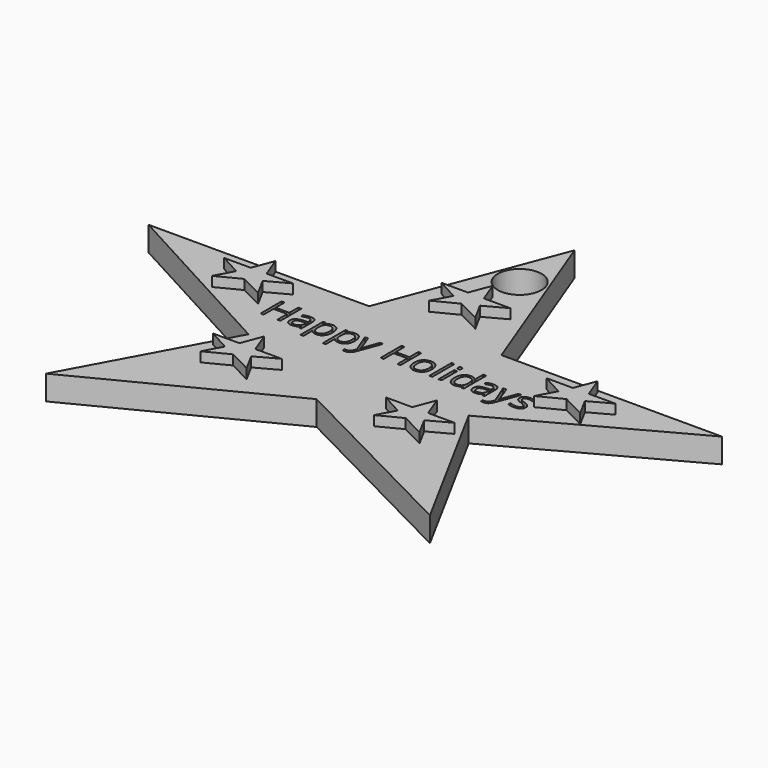
from build123d import *

# Parameters (mm, degrees)
F1_DEPTH     = 5
F2_TEXT_SIZE = 7.4632064853
F3_DEPTH     = 2.5
F4_R         = 4.4811489531
F5_DEPTH     = 25
F7_DEPTH     = 7


# Not quite as in the source:
# - Text() gives the source's letters only with a copy of the font that has no kerning and outlines rounded to 1/6400 em; it was checked with that copy


with BuildPart() as f1:
    # F0 (on Top) → F1 (new body)
    with BuildSketch(Plane.XY):
        Polygon((13.5034965324, 19.5594248276), (0, 55.0792162318), (-13.5034965324, 19.5594248276), (-58.5034965324, 19.5594248276), (-22.4697775957, 0), (-39.1668475705, -30.7604917753), (0, -10.71160025), (39.1668475705, -30.7604917753), (22.4697775957, 0), (58.5034965324, 19.5594248276), align=None)
    extrude(amount=F1_DEPTH)

    # F2 (on face) → F3 (cut)
    with BuildSketch(Plane.XY.offset(5)):
        with Locations((-26.1730113998, 6.8057645112)):
            Text('Happy Holidays', F2_TEXT_SIZE, font='Open Sans', text_align=(TextAlign.LEFT, TextAlign.BOTTOM))
    extrude(amount=-F3_DEPTH, mode=Mode.SUBTRACT)

    # F4 (on face) → F5 (cut)
    with BuildSketch(Plane.XY.offset(5)):
        with Locations((0, 41.0946980119)):
            Circle(F4_R)
    extrude(amount=-F5_DEPTH, mode=Mode.SUBTRACT)

    # F6 (on Top) → F7 (join)
    with BuildSketch(Plane.XY):
        Polygon((1.4968993236, 30.0896251639), (-0.1239613579, 34.3531604018), (-1.7448220394, 30.0896251639), (-7.146291984, 30.0896251639), (-2.8210686545, 27.7418552674), (-4.8252624685, 24.0495914495), (-0.1239613579, 26.4561133383), (4.5773397527, 24.0495914495), (2.5731459387, 27.7418552674), (6.8983692682, 30.0896251639), align=None)
        Polygon((-16.0245638686, -6.3085789717), (-17.6454245501, -2.0450437337), (-19.2662852316, -6.3085789717), (-24.6677551762, -6.3085789717), (-20.3425318467, -8.6563488681), (-22.3467256607, -12.348612686), (-17.6454245501, -9.9420907972), (-13, -12.320010356), (-14.9794849232, -8.6732669579), (-10.623093924, -6.3085789717), align=None)
        Polygon((19.2662843003, -6.3455471315), (17.6454236188, -2.0820118935), (16.0245629373, -6.3455471315), (10.6230929927, -6.3455471315), (14.9483163222, -8.6933170279), (13, -12.2826394837), (17.5728109542, -9.9418896793), (22.3467247294, -12.3855808459), (20.3425309154, -8.6933170279), (24.6677542449, -6.3455471315), align=None)
        Polygon((35.1189136321, 14.8292916444), (33.4980529506, 19.0928268824), (31.8771922691, 14.8292916444), (26.4757223244, 14.8292916444), (30.800945654, 12.481521748), (28.7967518399, 8.7892579301), (33.4980529506, 11.1957798189), (38.1993540612, 8.7892579301), (36.1951602471, 12.481521748), (40.5203835767, 14.8292916444), align=None)
        Polygon((-30.8826358509, 15.1366139896), (-32.5034965324, 19.4001492276), (-34.1243572139, 15.1366139896), (-39.5258271586, 15.1366139896), (-35.200603829, 12.7888440931), (-37.2047976431, 9.0965802752), (-32.5034965324, 11.503102164), (-27.8021954218, 9.0965802752), (-29.8063892359, 12.7888440931), (-25.4811659063, 15.1366139896), align=None)
    extrude(amount=F7_DEPTH)


solid = f1.part
